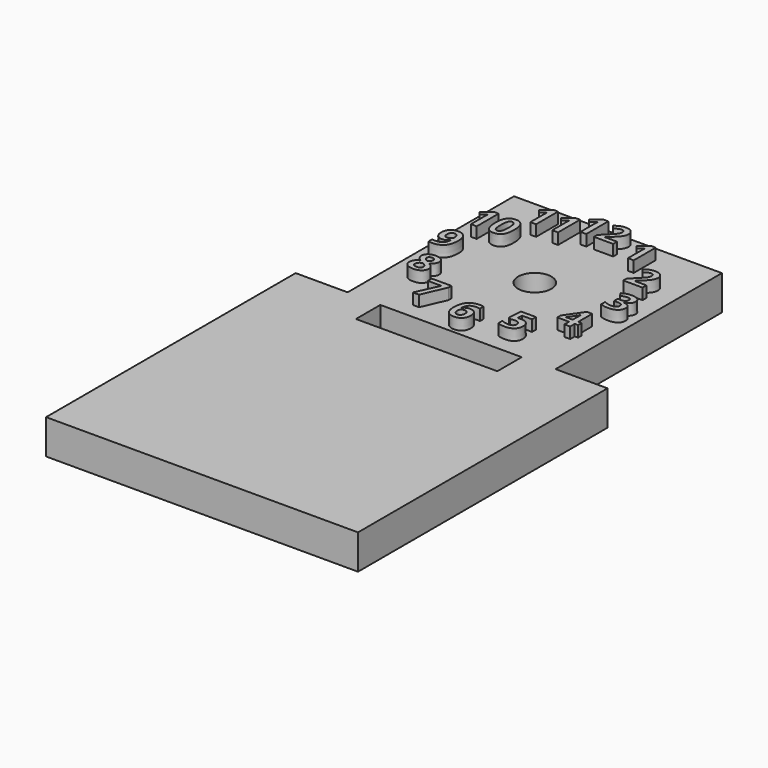
from build123d import *

# Parameters (mm, degrees)
F2_DEPTH     = 3.175
F3_W         = 12.954
F3_H         = 2.794
F4_DEPTH     = 25.4
F5_TEXT_SIZE = 3.5277777778
F6_DEPTH     = 1.016
F7_R         = 1.524
F8_DEPTH     = 3.175


# Not quite as in the source:
# - Text() gives the source's letters only with a copy of the font that has no kerning and outlines rounded to 1/6400 em; it was checked with that copy


with BuildPart() as f2:
    # F1 (on offset) → F2 (new body)
    with BuildSketch(Plane.XY):
        Polygon((-9.525, 14.2875), (-14.2875, 14.2875), (-14.2875, -14.2875), (14.2875, -14.2875), (14.2875, 14.2875), (9.525, 14.2875), (9.525, 33.3375), (-9.525, 33.3375), align=None)
    extrude(amount=F2_DEPTH)

    # F3 (on face) → F4 (cut)
    with BuildSketch(Plane.XY.offset(3.175)):
        with Locations((0, 12.827)):
            Rectangle(F3_W, F3_H)
    extrude(amount=-F4_DEPTH, mode=Mode.SUBTRACT)

    # F5 (on face) → F6 (join)
    with BuildSketch(Plane.XY.offset(3.175)):
        with Locations((3.1256662326, 29.4165766425)):
            Text('1', F5_TEXT_SIZE, font='Open Sans', font_style=FontStyle.BOLD, text_align=(TextAlign.LEFT, TextAlign.BOTTOM))
        with Locations((5.8088531182, 26.51125)):
            Text('2', F5_TEXT_SIZE, font='Open Sans', font_style=FontStyle.BOLD, text_align=(TextAlign.LEFT, TextAlign.BOTTOM))
        with Locations((6.8844032118, 22.5425)):
            Text('3', F5_TEXT_SIZE, font='Open Sans', font_style=FontStyle.BOLD, text_align=(TextAlign.LEFT, TextAlign.BOTTOM))
        with Locations((5.7804655314, 18.57375)):
            Text('4', F5_TEXT_SIZE, font='Open Sans', font_style=FontStyle.BOLD, text_align=(TextAlign.LEFT, TextAlign.BOTTOM))
        with Locations((2.9266775174, 15.6684233575)):
            Text('5', F5_TEXT_SIZE, font='Open Sans', font_style=FontStyle.BOLD, text_align=(TextAlign.LEFT, TextAlign.BOTTOM))
        with Locations((-1.0652235243, 14.605)):
            Text('6', F5_TEXT_SIZE, font='Open Sans', font_style=FontStyle.BOLD, text_align=(TextAlign.LEFT, TextAlign.BOTTOM))
        with Locations((-5.0339735243, 15.6684233575)):
            Text('7', F5_TEXT_SIZE, font='Open Sans', font_style=FontStyle.BOLD, text_align=(TextAlign.LEFT, TextAlign.BOTTOM))
        with Locations((-7.9340636217, 18.57375)):
            Text('8', F5_TEXT_SIZE, font='Open Sans', font_style=FontStyle.BOLD, text_align=(TextAlign.LEFT, TextAlign.BOTTOM))
        with Locations((-8.9974869792, 22.5425)):
            Text('9', F5_TEXT_SIZE, font='Open Sans', font_style=FontStyle.BOLD, text_align=(TextAlign.LEFT, TextAlign.BOTTOM))
        with Locations((-2.0720182292, 30.48)):
            Text('12', F5_TEXT_SIZE, font='Open Sans', font_style=FontStyle.BOLD, text_align=(TextAlign.LEFT, TextAlign.BOTTOM))
        with Locations((-5.8186284722, 29.4165766425)):
            Text('11', F5_TEXT_SIZE, font='Open Sans', font_style=FontStyle.BOLD, text_align=(TextAlign.LEFT, TextAlign.BOTTOM))
        with Locations((-8.9392046807, 26.51125)):
            Text('10', F5_TEXT_SIZE, font='Open Sans', font_style=FontStyle.BOLD, text_align=(TextAlign.LEFT, TextAlign.BOTTOM))
    extrude(amount=F6_DEPTH)

    # F7 (on face) → F8 (cut, through all)
    with BuildSketch(Plane.XY.offset(3.175)):
        with Locations((0, 23.8125)):
            Circle(F7_R)
    extrude(amount=-F8_DEPTH, mode=Mode.SUBTRACT)


solid = f2.part
